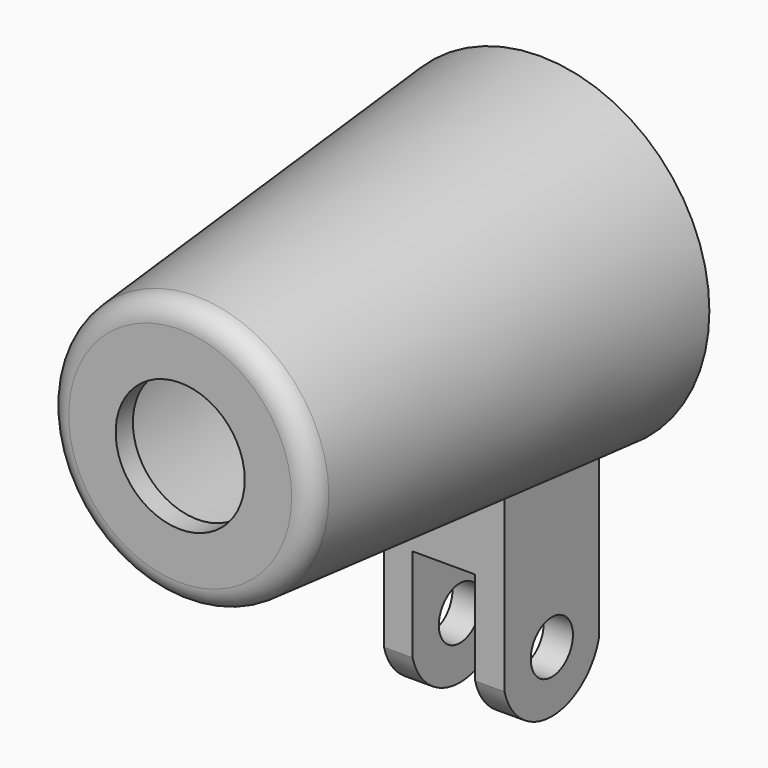
from build123d import *

# Parameters (mm, degrees)
F0_R      = 7.875
F2_R      = 6.1
F4_T      = -1
F5_R      = 3
F6_DEPTH  = 12.5
F7_R      = 1.225
F8_DEPTH  = 2.8
F9_W      = 2.908817606
F9_H      = 7.2918525926
F10_DEPTH = 20.9010001
F11_R     = 1


with BuildPart() as f3:
    # F0 (on Front) → F3 section 0
    with BuildSketch(Plane.XZ):
        Circle(F0_R)
    # F2 (on offset) → F3 section 1
    with BuildSketch(Plane.XZ.offset(20.9)):
        Circle(F2_R)
    loft()

    # F4
    f4_openings = [f3.faces().sort_by_distance(p)[0] for p in [
        (0, 0, 0),
    ]]
    offset(amount=F4_T, openings=f4_openings, kind=Kind.INTERSECTION)

    # F5 (on offset) → F6 (cut, symmetric)
    with BuildSketch(Plane.XZ.offset(20.9)):
        Circle(F5_R)
    extrude(amount=F6_DEPTH, both=True, mode=Mode.SUBTRACT)

    # F7 (on Right) → F8 (join, symmetric)
    with BuildSketch(Plane.YZ):
        with BuildLine():
            Line((-5.5590723408, -6.6040260717), (-5.5590723408, -14.9660339587))
            ThreePointArc((-5.5590723408, -14.9660339587), (-2.8090723408, -17.0962775531), (-0.0590723408, -14.9660339587))
            Line((-0.0590723408, -14.9660339587), (-0.0590723408, -7.0811193436))
            Line((-0.0590723408, -7.0811193436), (-5.5590723408, -6.6040260717))
        make_face()
        with Locations((-2.8090723408, -14.256124013)):
            Circle(F7_R, mode=Mode.SUBTRACT)
    extrude(amount=F8_DEPTH, both=True)

    # F9 (on offset) → F10 (cut, through all)
    with BuildSketch(Plane.XZ.offset(20.9)):
        with Locations((-0.016908803, -14.2587911789)):
            Rectangle(F9_W, F9_H)
    extrude(amount=-F10_DEPTH, mode=Mode.SUBTRACT)

    # F11
    f11_edges = [f3.edges().sort_by_distance(p)[0] for p in [
        (-6.1, -20.9, 0),
    ]]
    fillet(f11_edges, radius=F11_R)


solid = f3.part
